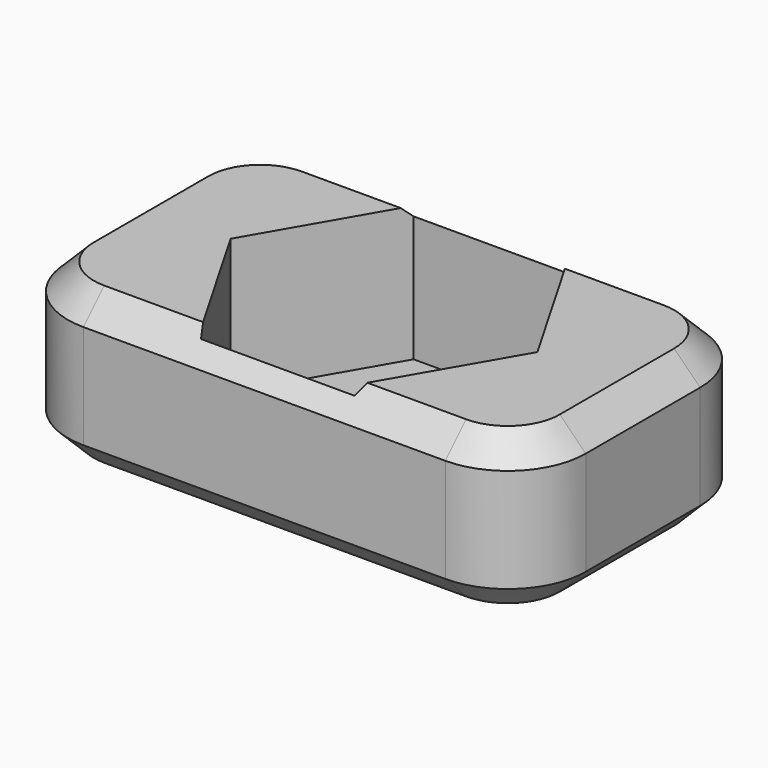
from build123d import *

# Parameters (mm, degrees)
F1_DEPTH     = 6
F3_DEPTH     = 5.2
F4_T1_DEPTH  = 13.92
F4_T3_DEPTH  = 5.5
F4_T6_ANGLE  = 90
F4_T8_ANGLE  = 90
F4_T10_ANGLE = 90
F4_T12_ANGLE = 90
F4_T14_ANGLE = 90
F4_T16_ANGLE = 90
F4_T18_ANGLE = 90
F4_T20_ANGLE = 90


# Not quite as in the source:
# - a fillet or chamfer that OpenCascade refuses, or shapes differently, is made with other operations: its cross-section is extruded or revolved along the edge and cut away or added


with BuildPart() as f1:
    # F0 (on Top) → F1 (new body)
    with BuildSketch(Plane.XY):
        with BuildLine():
            Line((6.96, 5.75), (-6.96, 5.75))
            ThreePointArc((-6.96, 5.75), (-9.0813203436, 4.8713203436), (-9.96, 2.75))
            Line((-9.96, 2.75), (-9.96, -2.75))
            ThreePointArc((-9.96, -2.75), (-9.0813203436, -4.8713203436), (-6.96, -5.75))
            Line((-6.96, -5.75), (6.96, -5.75))
            ThreePointArc((6.96, -5.75), (9.0813203436, -4.8713203436), (9.96, -2.75))
            Line((9.96, -2.75), (9.96, 2.75))
            ThreePointArc((9.96, 2.75), (9.0813203436, 4.8713203436), (6.96, 5.75))
        make_face()
    extrude(amount=F1_DEPTH)

    # F2 (on face) → F3 (cut)
    with BuildSketch(Plane.XY.offset(6)):
        Polygon((2.95, 5.1095498823), (-2.95, 5.1095498823), (-5.9, 0), (-2.95, -5.1095498823), (2.95, -5.1095498823), (5.9, 0), align=None)
    extrude(amount=-F3_DEPTH, mode=Mode.SUBTRACT)

    # F4: chamfer of 1 on 2 edges, made by hand

    # F4_s2 → F4_t1 (cut)
    with BuildSketch(Plane.YZ.offset(-6.96)):
        Polygon((5.75, 5), (4.75, 6), (5.75, 6), align=None)
        Polygon((5.75, 1), (4.75, 0), (5.75, 0), align=None)
        Polygon((-4.75, 0), (-5.75, 1), (-5.75, 0), align=None)
        Polygon((-4.75, 6), (-5.75, 5), (-5.75, 6), align=None)
    extrude(amount=F4_T1_DEPTH, mode=Mode.SUBTRACT)

    # F4_s4 → F4_t3 (cut)
    with BuildSketch(Plane.XZ.offset(-2.75)):
        Polygon((-8.96, 0), (-9.96, 1), (-9.96, 0), align=None)
        Polygon((8.96, 0), (9.96, 1), (9.96, 0), align=None)
        Polygon((-8.96, 6), (-9.96, 5), (-9.96, 6), align=None)
        Polygon((8.96, 6), (9.96, 5), (9.96, 6), align=None)
    extrude(amount=F4_T3_DEPTH, mode=Mode.SUBTRACT)

    # F4_s5 → F4_t6 (revolve, cut)
    with BuildSketch(Plane.XZ.offset(-2.75)):
        Polygon((9.96, 1), (8.96, 0), (9.96, 0), align=None)
    revolve(axis=Axis((6.96, 2.75, 0), (0, 0, 1)), revolution_arc=F4_T6_ANGLE, mode=Mode.SUBTRACT)

    # F4_s7 → F4_t8 (revolve, cut)
    with BuildSketch(Plane.YZ.offset(-6.96)):
        Polygon((5.75, 1), (4.75, 0), (5.75, 0), align=None)
    revolve(axis=Axis((-6.96, 2.75, 0), (0, 0, 1)), revolution_arc=F4_T8_ANGLE, mode=Mode.SUBTRACT)

    # F4_s9 → F4_t10 (revolve, cut)
    with BuildSketch(Plane.XZ.offset(2.75)):
        Polygon((-8.96, 0), (-9.96, 1), (-9.96, 0), align=None)
    revolve(axis=Axis((-6.96, -2.75, 0), (0, 0, 1)), revolution_arc=F4_T10_ANGLE, mode=Mode.SUBTRACT)

    # F4_s11 → F4_t12 (revolve, cut)
    with BuildSketch(Plane.YZ.offset(6.96)):
        Polygon((-4.75, 0), (-5.75, 1), (-5.75, 0), align=None)
    revolve(axis=Axis((6.96, -2.75, 0), (0, 0, 1)), revolution_arc=F4_T12_ANGLE, mode=Mode.SUBTRACT)

    # F4_s13 → F4_t14 (revolve, cut)
    with BuildSketch(Plane.XZ.offset(-2.75)):
        Polygon((9.96, 5), (8.96, 6), (9.96, 6), align=None)
    revolve(axis=Axis((6.96, 2.75, 6), (0, 0, 1)), revolution_arc=F4_T14_ANGLE, mode=Mode.SUBTRACT)

    # F4_s15 → F4_t16 (revolve, cut)
    with BuildSketch(Plane.YZ.offset(-6.96)):
        Polygon((5.75, 5), (4.75, 6), (5.75, 6), align=None)
    revolve(axis=Axis((-6.96, 2.75, 6), (0, 0, 1)), revolution_arc=F4_T16_ANGLE, mode=Mode.SUBTRACT)

    # F4_s17 → F4_t18 (revolve, cut)
    with BuildSketch(Plane.XZ.offset(2.75)):
        Polygon((-8.96, 6), (-9.96, 5), (-9.96, 6), align=None)
    revolve(axis=Axis((-6.96, -2.75, 6), (0, 0, 1)), revolution_arc=F4_T18_ANGLE, mode=Mode.SUBTRACT)

    # F4_s19 → F4_t20 (revolve, cut)
    with BuildSketch(Plane.YZ.offset(6.96)):
        Polygon((-4.75, 6), (-5.75, 5), (-5.75, 6), align=None)
    revolve(axis=Axis((6.96, -2.75, 6), (0, 0, 1)), revolution_arc=F4_T20_ANGLE, mode=Mode.SUBTRACT)


solid = f1.part
